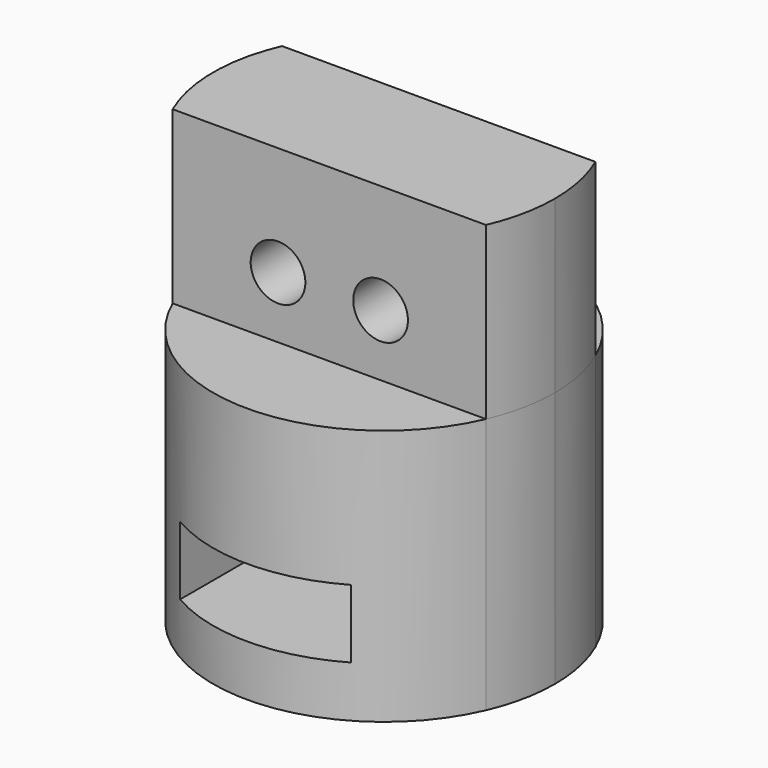
from build123d import *
from build123d import SkipClean  # not in build123d's __all__

# Parameters (mm, degrees)
F0_R     = 1.5
F1_DEPTH = 15
F3_W     = 10
F3_H     = 4
F5_DEPTH = 45.85
F6_DEPTH = 10
F7_R     = 1.6
F8_DEPTH = 14.001


# Not quite as in the source:
# - after a boolean that leaves OpenCascade's solid faulty, fix() repairs it


with BuildPart() as f1:
    # F0 (on Top) → F1 (new body)
    with BuildSketch(Plane.XY):
        with BuildLine():
            ThreePointArc((9.1651513899, -4), (9.7890631293, -2.0430964369), (10, 0))
            ThreePointArc((10, 0), (9.7890631293, 2.0430964369), (9.1651513899, 4))
            Line((9.1651513899, 4), (-9.1651513899, 4))
            ThreePointArc((-9.1651513899, 4), (-10, 0), (-9.1651513899, -4))
            Line((-9.1651513899, -4), (9.1651513899, -4))
        make_face()
        Circle(F0_R, mode=Mode.SUBTRACT)
        with BuildLine():
            ThreePointArc((-9.1651513899, -4), (0, -10), (9.1651513899, -4))
            Line((9.1651513899, -4), (-9.1651513899, -4))
        make_face()
        with BuildLine():
            Line((-9.1651513899, 4), (9.1651513899, 4))
            ThreePointArc((9.1651513899, 4), (0, 10), (-9.1651513899, 4))
        make_face()
    extrude(amount=-F1_DEPTH)

    # F3 (on offset) → F5 (cut, through all)
    with BuildSketch(Plane.XZ.offset(40)):
        with Locations((0, -10)):
            Rectangle(F3_W, F3_H)
    extrude(amount=-F5_DEPTH, mode=Mode.SUBTRACT)

    # F0 (on Top) → F6 (join)
    with BuildSketch(Plane.XY):
        with BuildLine():
            ThreePointArc((9.1651513899, -4), (9.7890631293, -2.0430964369), (10, 0))
            ThreePointArc((10, 0), (9.7890631293, 2.0430964369), (9.1651513899, 4))
            Line((9.1651513899, 4), (-9.1651513899, 4))
            ThreePointArc((-9.1651513899, 4), (-10, 0), (-9.1651513899, -4))
            Line((-9.1651513899, -4), (9.1651513899, -4))
        make_face()
        Circle(F0_R, mode=Mode.SUBTRACT)
        Circle(F0_R)
    with SkipClean():  # cleaning this boolean's faces spoils the solid; the shape is the same uncleaned
        extrude(amount=F6_DEPTH)

    # F7 (on face) → F8 (cut, through all)
    with BuildSketch(Plane.XZ.offset(4)):
        with Locations((-3, 3.6)):
            Circle(F7_R)
        with Locations((3, 3.6)):
            Circle(F7_R)
    extrude(amount=-F8_DEPTH, mode=Mode.SUBTRACT)

    add(f1.part.fix(), mode=Mode.REPLACE)


solid = f1.part
